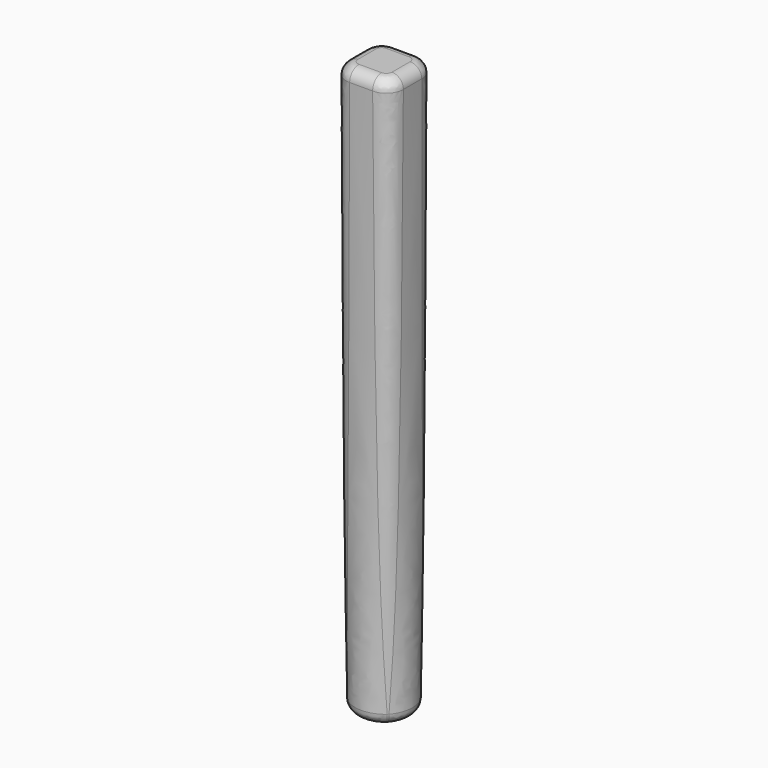
from build123d import *

# Parameters (mm, degrees)
F1_W = 50
F1_H = 50
F4_R = 15
F5_R = 10


# Not quite as in the source:
# - the arcs of a loft's sections are written as splines that run evenly, so that the points pair up as in the source's solid


with BuildPart() as f3:
    # F1 (on offset) → F3 section 0
    with BuildSketch(Plane.XY.offset(500)):
        Rectangle(F1_W, F1_H)
    # F2 (on Top) → F3 section 1
    with BuildSketch(Plane.XY):
        with BuildLine():
            add(Edge.make_bspline(
                [(17.6776695297, -17.6776695297), (18.8346702948, -16.5206687645), (19.8776906395, -15.2497447972), (21.6957899756, -12.5287668538), (22.4708240108, -11.0787801592), (23.7231526147, -8.0553914591), (24.2004162171, -6.4820642127), (24.838847803, -3.2724518881), (25, -1.6362461737), (25, 1.6362461737), (24.838847803, 3.2724518881), (24.2004162171, 6.4820642127), (23.7231526147, 8.0553914591), (22.4708240108, 11.0787801592), (21.6957899756, 12.5287668538), (19.8776906395, 15.2497447972), (18.8346702948, 16.5206687645), (17.6776695297, 17.6776695297)],
                knots=[0, 0, 0, 0, 0.125, 0.125, 0.25, 0.25, 0.375, 0.375, 0.5, 0.5, 0.625, 0.625, 0.75, 0.75, 0.875, 0.875, 1, 1, 1, 1], degree=3))
            add(Edge.make_bspline(
                [(17.6776695297, 17.6776695297), (16.5206687645, 18.8346702948), (15.2497447972, 19.8776906395), (12.5287668538, 21.6957899756), (11.0787801592, 22.4708240108), (8.0553914591, 23.7231526147), (6.4820642127, 24.2004162171), (3.2724518881, 24.838847803), (1.6362461737, 25), (-1.6362461737, 25), (-3.2724518881, 24.838847803), (-6.4820642127, 24.2004162171), (-8.0553914591, 23.7231526147), (-11.0787801592, 22.4708240108), (-12.5287668538, 21.6957899756), (-15.2497447972, 19.8776906395), (-16.5206687645, 18.8346702948), (-17.6776695297, 17.6776695297)],
                knots=[0, 0, 0, 0, 0.125, 0.125, 0.25, 0.25, 0.375, 0.375, 0.5, 0.5, 0.625, 0.625, 0.75, 0.75, 0.875, 0.875, 1, 1, 1, 1], degree=3))
            add(Edge.make_bspline(
                [(-17.6776695297, 17.6776695297), (-18.8346702948, 16.5206687645), (-19.8776906395, 15.2497447972), (-21.6957899756, 12.5287668538), (-22.4708240108, 11.0787801592), (-23.7231526147, 8.0553914591), (-24.2004162171, 6.4820642127), (-24.838847803, 3.2724518881), (-25, 1.6362461737), (-25, -1.6362461737), (-24.838847803, -3.2724518881), (-24.2004162171, -6.4820642127), (-23.7231526147, -8.0553914591), (-22.4708240108, -11.0787801592), (-21.6957899756, -12.5287668538), (-19.8776906395, -15.2497447972), (-18.8346702948, -16.5206687645), (-17.6776695297, -17.6776695297)],
                knots=[0, 0, 0, 0, 0.125, 0.125, 0.25, 0.25, 0.375, 0.375, 0.5, 0.5, 0.625, 0.625, 0.75, 0.75, 0.875, 0.875, 1, 1, 1, 1], degree=3))
            add(Edge.make_bspline(
                [(-17.6776695297, -17.6776695297), (-16.5206687645, -18.8346702948), (-15.2497447972, -19.8776906395), (-12.5287668538, -21.6957899756), (-11.0787801592, -22.4708240108), (-8.0553914591, -23.7231526147), (-6.4820642127, -24.2004162171), (-3.2724518881, -24.838847803), (-1.6362461737, -25), (1.6362461737, -25), (3.2724518881, -24.838847803), (6.4820642127, -24.2004162171), (8.0553914591, -23.7231526147), (11.0787801592, -22.4708240108), (12.5287668538, -21.6957899756), (15.2497447972, -19.8776906395), (16.5206687645, -18.8346702948), (17.6776695297, -17.6776695297)],
                knots=[0, 0, 0, 0, 0.125, 0.125, 0.25, 0.25, 0.375, 0.375, 0.5, 0.5, 0.625, 0.625, 0.75, 0.75, 0.875, 0.875, 1, 1, 1, 1], degree=3))
        make_face()
    loft(ruled=True)

    # F4
    f4_edges = [f3.edges().sort_by_distance(p)[0] for p in [
        (21.338835, 21.338835, 250),
        (21.338835, -21.338835, 250),
        (-21.338835, 21.338835, 250),
        (-21.338835, -21.338835, 250),
    ]]
    fillet(f4_edges, radius=F4_R)

    # F5
    f5_edges = [f3.edges().sort_by_distance(p)[0] for p in [
        (25, 0, 500),
        (23.884724, -11.932761, 249.916263),
        (23.884723, 11.932762, 249.916196),
        (25, 0, 0),
        (0, 25, 500),
        (11.932761, 23.884724, 249.916258),
        (-11.932761, 23.884724, 249.916268),
        (0, 25, 0),
        (-25, 0, 500),
        (-23.884723, 11.932762, 249.916196),
        (-23.884724, -11.932761, 249.916269),
        (-25, 0, 0),
        (0, -25, 500),
        (-11.932762, -23.884723, 249.916196),
        (11.932762, -23.884723, 249.916196),
        (0, -25, 0),
        (20.606159, -20.606159, 500),
        (20.606159, 20.606159, 500),
        (-20.606159, -20.606159, 500),
        (-20.606159, 20.606159, 500),
    ]]
    fillet(f5_edges, radius=F5_R)


solid = f3.part
